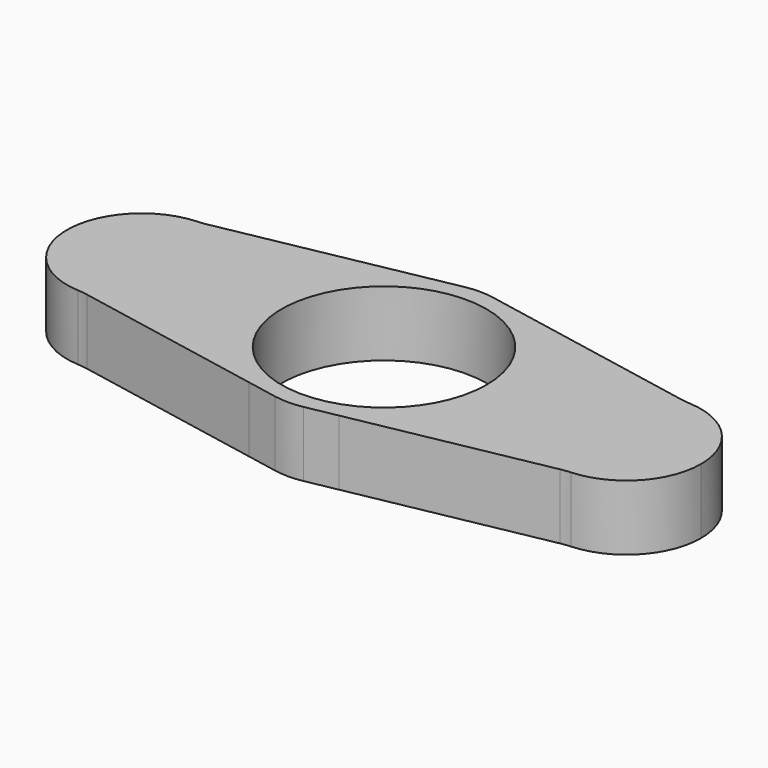
from build123d import *

# Parameters (mm, degrees)
F0_R     = 11
F1_DEPTH = 7
F2_R     = 8
F3_R     = 8


with BuildPart() as f1:
    # F0 (on Top) → F1 (new body)
    with BuildSketch(Plane.XY):
        with BuildLine():
            ThreePointArc((4.8216833096, -12.0727532097), (10.7629429763, -7.2910258872), (13, 0))
            ThreePointArc((13, 0), (10.7629429763, 7.2910258872), (4.8216833096, 12.0727532097))
            Line((4.8216833096, 12.0727532097), (0, 13))
            Line((0, 13), (-4.8216833096, 12.0727532097))
            ThreePointArc((-4.8216833096, 12.0727532097), (-13, 0), (-4.8216833096, -12.0727532097))
            Line((-4.8216833096, -12.0727532097), (0, -13))
            Line((0, -13), (4.8216833096, -12.0727532097))
        make_face()
        Circle(F0_R, mode=Mode.SUBTRACT)
        with BuildLine():
            ThreePointArc((4.8216833096, 12.0727532097), (10.7629429763, 7.2910258872), (13, 0))
            ThreePointArc((13, 0), (10.7629429763, -7.2910258872), (4.8216833096, -12.0727532097))
            Line((4.8216833096, -12.0727532097), (26, -8))
            ThreePointArc((26, -8), (18, 0), (26, 8))
            Line((26, 8), (4.8216833096, 12.0727532097))
        make_face()
        with BuildLine():
            ThreePointArc((34, 0), (31.6568542495, 5.6568542495), (26, 8))
            ThreePointArc((26, 8), (18, 0), (26, -8))
            ThreePointArc((26, -8), (31.6568542495, -5.6568542495), (34, 0))
        make_face()
        with BuildLine():
            ThreePointArc((-4.8216833096, -12.0727532097), (-13, 0), (-4.8216833096, 12.0727532097))
            Line((-4.8216833096, 12.0727532097), (-26, 8))
            ThreePointArc((-26, 8), (-20.3431457505, 5.6568542495), (-18, 0))
            ThreePointArc((-18, 0), (-20.3431457505, -5.6568542495), (-26, -8))
            Line((-26, -8), (-4.8216833096, -12.0727532097))
        make_face()
        with BuildLine():
            ThreePointArc((-18, 0), (-20.3431457505, 5.6568542495), (-26, 8))
            ThreePointArc((-26, 8), (-34, 0), (-26, -8))
            ThreePointArc((-26, -8), (-20.3431457505, -5.6568542495), (-18, 0))
        make_face()
    extrude(amount=F1_DEPTH)

    # F2
    f2_edges = [f1.edges().sort_by_distance(p)[0] for p in [
        (0, -13, 3.5),
        (0, 13, 3.5),
    ]]
    fillet(f2_edges, radius=F2_R)

    # F3
    f3_edges = [f1.edges().sort_by_distance(p)[0] for p in [
        (-26, -8, 3.5),
        (-26, 8, 3.5),
        (26, 8, 3.5),
        (26, -8, 3.5),
    ]]
    fillet(f3_edges, radius=F3_R)


solid = f1.part
